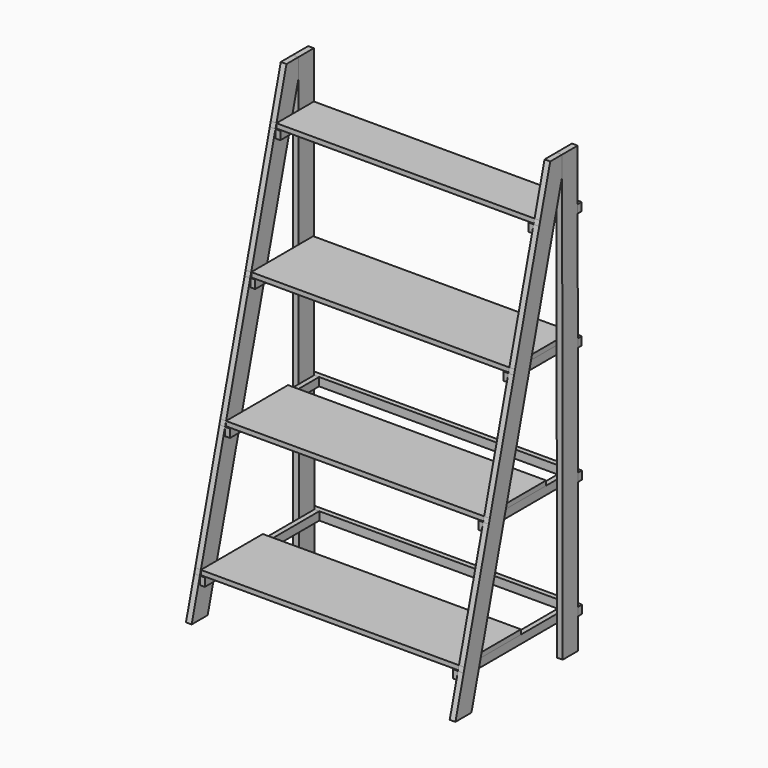
from build123d import *

# Parameters (mm, degrees)
F1_DEPTH      = 11
F1_DEPTH_BACK = 11
F0_W          = 75
F0_H          = 18
F0_H_2        = 32
F0_W_2        = 70.9380639768
F0_H_3        = 426.0930354319
F0_H_4        = 118
F2_DEPTH      = 11
F2_DEPTH_BACK = 11
F5_DEPTH      = 19
F8_DEPTH      = 500
F8_DEPTH_BACK = 500
F10_DEPTH     = 19
F12_ANGLE     = 180


# Not quite as in the source:
# - a feature names something its author has since deleted; it is built from what else it names


with BuildPart() as f1:
    # F0 (on Right) → F1 (new body, two sides)
    with BuildSketch(Plane.YZ) as f1_sk:
        Polygon((183.8850214869, 172.046517716), (183.8850214869, 204.046517716), (179.0619360232, 204.046517716), (106.2393079562, 204.046517716), (114.813682114, 172.046517716), align=None)
        Polygon((301.8075949255, -236.046517716), (183.8850214869, 204.046517716), (183.8850214869, 172.046517716), (114.813682114, 172.046517716), (224.1618813947, -236.046517716), align=None)
        Polygon((183.8850214869, 204.046517716), (179.0619360232, 222.046517716), (179.0619360232, 204.046517716), align=None)
        Polygon((179.0619360232, 204.046517716), (179.0619360232, 222.046517716), (101.4162224924, 222.046517716), (106.2393079562, 204.046517716), align=None)
        Polygon((179.0619360232, 222.046517716), (61.1393625846, 662.1395531479), (61.1393625846, 630.1395531479), (-7.9319767883, 630.1395531479), (101.4162224924, 222.046517716), align=None)
        Polygon((424.5532538278, -694.1395531479), (306.6306803892, -254.046517716), (306.6306803892, -286.046517716), (237.5593410163, -286.046517716), (346.907540297, -694.1395531479), align=None)
        Polygon((306.6306803892, -286.046517716), (306.6306803892, -254.046517716), (301.8075949255, -254.046517716), (228.9849668585, -254.046517716), (237.5593410163, -286.046517716), align=None)
        Polygon((301.8075949255, -254.046517716), (301.8075949255, -236.046517716), (224.1618813947, -236.046517716), (228.9849668585, -254.046517716), align=None)
        Polygon((306.6306803892, -254.046517716), (301.8075949255, -236.046517716), (301.8075949255, -254.046517716), align=None)
        Polygon((469.5687181562, -862.1395531479), (429.3763392916, -712.1395531479), (429.3763392915, -744.1395531479), (360.3049999186, -744.1395531479), (391.9230046255, -862.1395531479), align=None)
        Polygon((429.3763392915, -744.1395531479), (429.3763392915, -712.1395531479), (424.5532538278, -712.1395531479), (351.7306257608, -712.1395531479), (360.3049999186, -744.1395531479), align=None)
        Polygon((424.5532538278, -712.1395531479), (424.5532538278, -694.1395531479), (346.907540297, -694.1395531479), (351.7306257608, -712.1395531479), align=None)
        Polygon((429.3763392916, -712.1395531479), (424.5532538278, -694.1395531479), (424.5532538278, -712.1395531479), align=None)
        Polygon((7.5495240984, 862.1395531479), (-50, 862.1395531479), (-50, 787.1395531479), (-21.3294364099, 680.1395531479), (56.3162771209, 680.1395531479), align=None)
        Polygon((56.3162771209, 680.1395531479), (-21.3294364099, 680.1395531479), (-16.5063509461, 662.1395531479), (56.3162771209, 662.1395531479), align=None)
        Polygon((56.3162771209, 662.1395531479), (-16.5063509461, 662.1395531479), (-7.9319767883, 630.1395531479), (61.1393625846, 630.1395531479), (61.1393625846, 662.1395531479), align=None)
        Polygon((61.1393625846, 662.1395531479), (56.3162771209, 680.1395531479), (56.3162771209, 662.1395531479), align=None)
    extrude(amount=F1_DEPTH)
    extrude(f1_sk.sketch, amount=-F1_DEPTH_BACK)


with BuildPart() as f2:
    # F0 (on Right) → F2 (new body, two sides)
    with BuildSketch(Plane.YZ) as f2_sk:
        Polygon((-50, 862.1395531479), (-125, 862.1395531479), (-125, 680.1395531479), (-50, 680.1395531479), (-50, 787.1395531479), align=None)
        with Locations((-87.5, 671.1395531479)):
            Rectangle(F0_W, F0_H)
        Polygon((-50, 630.1395531479), (-125, 630.1395531479), (-125, 204.046517716), (-120.9380639768, 204.046517716), (-120.9380639768, 222.046517716), (-50, 222.046517716), align=None)
        with Locations((-87.5, 646.1395531479)):
            Rectangle(F0_W, F0_H_2)
        Polygon((-120.9380639768, 204.046517716), (-125, 204.046517716), (-125, 172.046517716), (-50, 172.046517716), (-50, 204.046517716), align=None)
        with Locations((-85.4690319884, 213.046517716)):
            Rectangle(F0_W_2, F0_H)
        with Locations((-87.5, -41)):
            Rectangle(F0_W, F0_H_3)
        with Locations((-87.5, -270.046517716)):
            Rectangle(F0_W, F0_H_2)
        with Locations((-87.5, -499.0930354319)):
            Rectangle(F0_W, F0_H_3)
        with Locations((-87.5, -728.1395531479)):
            Rectangle(F0_W, F0_H_2)
        with Locations((-87.5, -803.1395531479)):
            Rectangle(F0_W, F0_H_4)
    extrude(amount=F2_DEPTH)
    extrude(f2_sk.sketch, amount=-F2_DEPTH_BACK)


with BuildPart() as f1_1:
    # F3: moved
    add(f1.part.moved(Location((511, 0, 0))))


with BuildPart() as f2_1:
    # F3: moved
    add(f2.part.moved(Location((511, 0, 0))))


with BuildPart() as f4_1:
    # F4: copy of F1
    add(f1_1.part.moved(Location((-1022, 0, 0))))


with BuildPart() as f4_2:
    # F4: copy of F2
    add(f2_1.part.moved(Location((-1022, 0, 0))))


with BuildPart() as f5:
    # F0 (on Right) → F5 (new body)
    with BuildSketch(Plane.YZ):
        Polygon((124.5532538278, -712.1395531479), (-50, -712.1395531479), (-50, -744.1395531479), (360.3049999186, -744.1395531479), (351.7306257608, -712.1395531479), align=None)
        with Locations((-87.5, -728.1395531479)):
            Rectangle(F0_W, F0_H_2)
        Polygon((429.3763392915, -744.1395531479), (429.3763392915, -712.1395531479), (424.5532538278, -712.1395531479), (351.7306257608, -712.1395531479), (360.3049999186, -744.1395531479), align=None)
    extrude(amount=F5_DEPTH)


with BuildPart() as f5b:
    # F0 (on Right) → F5, piece 2 (new body)
    with BuildSketch(Plane.YZ):
        Polygon((306.6306803892, -286.046517716), (306.6306803892, -254.046517716), (301.8075949255, -254.046517716), (228.9849668585, -254.046517716), (237.5593410163, -286.046517716), align=None)
        Polygon((1.8075949255, -254.046517716), (-50, -254.046517716), (-50, -286.046517716), (237.5593410163, -286.046517716), (228.9849668585, -254.046517716), align=None)
        with Locations((-87.5, -270.046517716)):
            Rectangle(F0_W, F0_H_2)
    extrude(amount=F5_DEPTH)


with BuildPart() as f5c:
    # F0 (on Right) → F5, piece 3 (new body)
    with BuildSketch(Plane.YZ):
        Polygon((-120.9380639768, 204.046517716), (-125, 204.046517716), (-125, 172.046517716), (-50, 172.046517716), (-50, 204.046517716), align=None)
        Polygon((-50, 204.046517716), (-50, 172.046517716), (114.813682114, 172.046517716), (106.2393079562, 204.046517716), align=None)
        Polygon((183.8850214869, 172.046517716), (183.8850214869, 204.046517716), (179.0619360232, 204.046517716), (106.2393079562, 204.046517716), (114.813682114, 172.046517716), align=None)
    extrude(amount=F5_DEPTH)


with BuildPart() as f5d:
    # F0 (on Right) → F5, piece 4 (new body)
    with BuildSketch(Plane.YZ):
        with Locations((-87.5, 646.1395531479)):
            Rectangle(F0_W, F0_H_2)
        Polygon((-16.5063509461, 662.1395531479), (-50, 662.1395531479), (-50, 630.1395531479), (-7.9319767883, 630.1395531479), align=None)
        Polygon((56.3162771209, 662.1395531479), (-16.5063509461, 662.1395531479), (-7.9319767883, 630.1395531479), (61.1393625846, 630.1395531479), (61.1393625846, 662.1395531479), align=None)
    extrude(amount=F5_DEPTH)


with BuildPart() as f5d_1:
    # F6: moved
    add(f5d.part.moved(Location((-500, 0, 0))))


with BuildPart() as f5c_1:
    # F6: moved
    add(f5c.part.moved(Location((-500, 0, 0))))


with BuildPart() as f5b_1:
    # F6: moved
    add(f5b.part.moved(Location((-500, 0, 0))))


with BuildPart() as f5_1:
    # F6: moved
    add(f5.part.moved(Location((-500, 0, 0))))


with BuildPart() as f7_1:
    # F7: copy of F5c
    add(f5c_1.part.moved(Location((981, 0, 0))))


with BuildPart() as f7_2:
    # F7: copy of F5d
    add(f5d_1.part.moved(Location((981, 0, 0))))


with BuildPart() as f7_3:
    # F7: copy of F5b
    add(f5b_1.part.moved(Location((981, 0, 0))))


with BuildPart() as f7_4:
    # F7: copy of F5
    add(f5_1.part.moved(Location((981, 0, 0))))


with BuildPart() as f8:
    # F0 (on Right) → F8 (new body, two sides)
    with BuildSketch(Plane.YZ) as f8_sk:
        Polygon((-21.3294364099, 680.1395531479), (-50, 680.1395531479), (-50, 662.1395531479), (-16.5063509461, 662.1395531479), align=None)
        with Locations((-87.5, 671.1395531479)):
            Rectangle(F0_W, F0_H)
        Polygon((56.3162771209, 680.1395531479), (-21.3294364099, 680.1395531479), (-16.5063509461, 662.1395531479), (56.3162771209, 662.1395531479), align=None)
    extrude(amount=F8_DEPTH)
    extrude(f8_sk.sketch, amount=-F8_DEPTH_BACK)


with BuildPart() as f8b:
    # F0 (on Right) → F8, piece 2 (new body, two sides)
    with BuildSketch(Plane.YZ) as f8_2_sk:
        Polygon((179.0619360232, 204.046517716), (179.0619360232, 222.046517716), (101.4162224924, 222.046517716), (106.2393079562, 204.046517716), align=None)
        Polygon((101.4162224924, 222.046517716), (-50, 222.046517716), (-50, 204.046517716), (106.2393079562, 204.046517716), align=None)
        with Locations((-85.4690319884, 213.046517716)):
            Rectangle(F0_W_2, F0_H)
    extrude(amount=F8_DEPTH)
    extrude(f8_2_sk.sketch, amount=-F8_DEPTH_BACK)


with BuildPart() as f8c:
    # F0 (on Right) → F8, piece 3 (new body, two sides)
    with BuildSketch(Plane.YZ) as f8_3_sk:
        Polygon((228.9849668585, -254.046517716), (224.1618813947, -236.046517716), (1.8075949255, -236.046517716), (1.8075949255, -254.046517716), align=None)
        Polygon((301.8075949255, -254.046517716), (301.8075949255, -236.046517716), (224.1618813947, -236.046517716), (228.9849668585, -254.046517716), align=None)
    extrude(amount=F8_DEPTH)
    extrude(f8_3_sk.sketch, amount=-F8_DEPTH_BACK)


with BuildPart() as f8d:
    # F0 (on Right) → F8, piece 4 (new body, two sides)
    with BuildSketch(Plane.YZ) as f8_4_sk:
        Polygon((351.7306257608, -712.1395531479), (346.907540297, -694.1395531479), (124.5532538278, -694.1395531479), (124.5532538278, -712.1395531479), align=None)
        Polygon((424.5532538278, -712.1395531479), (424.5532538278, -694.1395531479), (346.907540297, -694.1395531479), (351.7306257608, -712.1395531479), align=None)
    extrude(amount=F8_DEPTH)
    extrude(f8_4_sk.sketch, amount=-F8_DEPTH_BACK)


with BuildPart() as f10:
    # F9 (on Front) → F10 (new body)
    with BuildSketch(Plane.XZ):
        Polygon((522, 630.139555), (522, 662.139555), (-522, 662.139555), (-522, 630.139555), (-442.7915117324, 630.139555), align=None)
    extrude(amount=F10_DEPTH)


with BuildPart() as f10b:
    # F9 (on Front) → F10, piece 2 (new body)
    with BuildSketch(Plane.XZ):
        Polygon((522, -712.139555), (442.7915117324, -712.139555), (-522, -712.139555), (-522, -744.139555), (522, -744.139555), align=None)
    extrude(amount=F10_DEPTH)


with BuildPart() as f10c:
    # F9 (on Front) → F10, piece 3 (new body)
    with BuildSketch(Plane.XZ):
        Polygon((522, 204.0465183333), (442.7915117324, 204.0465183333), (-522, 204.0465183333), (-522, 172.0465183333), (442.7915117324, 172.0465183333), (522, 172.0465183333), align=None)
    extrude(amount=F10_DEPTH)


with BuildPart() as f10d:
    # F9 (on Front) → F10, piece 4 (new body)
    with BuildSketch(Plane.XZ):
        Polygon((522, -254.0465183333), (-442.7915117324, -254.0465183333), (-522, -254.0465183333), (-522, -286.0465183333), (-442.7915117324, -286.0465183333), (522, -286.0465183333), align=None)
    extrude(amount=F10_DEPTH)


with BuildPart() as f10_1:
    # F11: moved
    add(f10.part.moved(Location((0, -125, 0))))


with BuildPart() as f10c_1:
    # F11: moved
    add(f10c.part.moved(Location((0, -125, 0))))


with BuildPart() as f10d_1:
    # F11: moved
    add(f10d.part.moved(Location((0, -125, 0))))


with BuildPart() as f10b_1:
    # F11: moved
    add(f10b.part.moved(Location((0, -125, 0))))


with BuildPart() as f1_2:
    # F12: moved
    add(f1_1.part.rotate(Axis((0, 0.9037974627, -15.0293707848), (0, 0.0008007353, -0.9999996794)), F12_ANGLE))


with BuildPart() as f2_2:
    # F12: moved
    add(f2_1.part.rotate(Axis((0, 0.9037974627, -15.0293707848), (0, 0.0008007353, -0.9999996794)), F12_ANGLE))


with BuildPart() as f4_1_1:
    # F12: moved
    add(f4_1.part.rotate(Axis((0, 0.9037974627, -15.0293707848), (0, 0.0008007353, -0.9999996794)), F12_ANGLE))


with BuildPart() as f4_2_1:
    # F12: moved
    add(f4_2.part.rotate(Axis((0, 0.9037974627, -15.0293707848), (0, 0.0008007353, -0.9999996794)), F12_ANGLE))


with BuildPart() as f5_2:
    # F12: moved
    add(f5_1.part.rotate(Axis((0, 0.9037974627, -15.0293707848), (0, 0.0008007353, -0.9999996794)), F12_ANGLE))


with BuildPart() as f5b_2:
    # F12: moved
    add(f5b_1.part.rotate(Axis((0, 0.9037974627, -15.0293707848), (0, 0.0008007353, -0.9999996794)), F12_ANGLE))


with BuildPart() as f7_4_1:
    # F12: moved
    add(f7_4.part.rotate(Axis((0, 0.9037974627, -15.0293707848), (0, 0.0008007353, -0.9999996794)), F12_ANGLE))


with BuildPart() as f5d_2:
    # F12: moved
    add(f5d_1.part.rotate(Axis((0, 0.9037974627, -15.0293707848), (0, 0.0008007353, -0.9999996794)), F12_ANGLE))


with BuildPart() as f7_3_1:
    # F12: moved
    add(f7_3.part.rotate(Axis((0, 0.9037974627, -15.0293707848), (0, 0.0008007353, -0.9999996794)), F12_ANGLE))


with BuildPart() as f7_1_1:
    # F12: moved
    add(f7_1.part.rotate(Axis((0, 0.9037974627, -15.0293707848), (0, 0.0008007353, -0.9999996794)), F12_ANGLE))


with BuildPart() as f8d_1:
    # F12: moved
    add(f8d.part.rotate(Axis((0, 0.9037974627, -15.0293707848), (0, 0.0008007353, -0.9999996794)), F12_ANGLE))


with BuildPart() as f7_2_1:
    # F12: moved
    add(f7_2.part.rotate(Axis((0, 0.9037974627, -15.0293707848), (0, 0.0008007353, -0.9999996794)), F12_ANGLE))


with BuildPart() as f8c_1:
    # F12: moved
    add(f8c.part.rotate(Axis((0, 0.9037974627, -15.0293707848), (0, 0.0008007353, -0.9999996794)), F12_ANGLE))


with BuildPart() as f8b_1:
    # F12: moved
    add(f8b.part.rotate(Axis((0, 0.9037974627, -15.0293707848), (0, 0.0008007353, -0.9999996794)), F12_ANGLE))


with BuildPart() as f8_1:
    # F12: moved
    add(f8.part.rotate(Axis((0, 0.9037974627, -15.0293707848), (0, 0.0008007353, -0.9999996794)), F12_ANGLE))


with BuildPart() as f10_2:
    # F12: moved
    add(f10_1.part.rotate(Axis((0, 0.9037974627, -15.0293707848), (0, 0.0008007353, -0.9999996794)), F12_ANGLE))


with BuildPart() as f10c_2:
    # F12: moved
    add(f10c_1.part.rotate(Axis((0, 0.9037974627, -15.0293707848), (0, 0.0008007353, -0.9999996794)), F12_ANGLE))


with BuildPart() as f10b_2:
    # F12: moved
    add(f10b_1.part.rotate(Axis((0, 0.9037974627, -15.0293707848), (0, 0.0008007353, -0.9999996794)), F12_ANGLE))


with BuildPart() as f10d_2:
    # F12: moved
    add(f10d_1.part.rotate(Axis((0, 0.9037974627, -15.0293707848), (0, 0.0008007353, -0.9999996794)), F12_ANGLE))


with BuildPart() as f5c_2:
    # F12: moved
    add(f5c_1.part.rotate(Axis((0, 0.9037974627, -15.0293707848), (0, 0.0008007353, -0.9999996794)), F12_ANGLE))


solid = Compound([f1_2.part, f2_2.part, f4_1_1.part, f4_2_1.part, f5_2.part, f5b_2.part, f7_4_1.part, f5d_2.part, f7_3_1.part, f7_1_1.part, f8d_1.part, f7_2_1.part, f8c_1.part, f8b_1.part, f8_1.part, f10_2.part, f10c_2.part, f10b_2.part, f10d_2.part, f5c_2.part])
